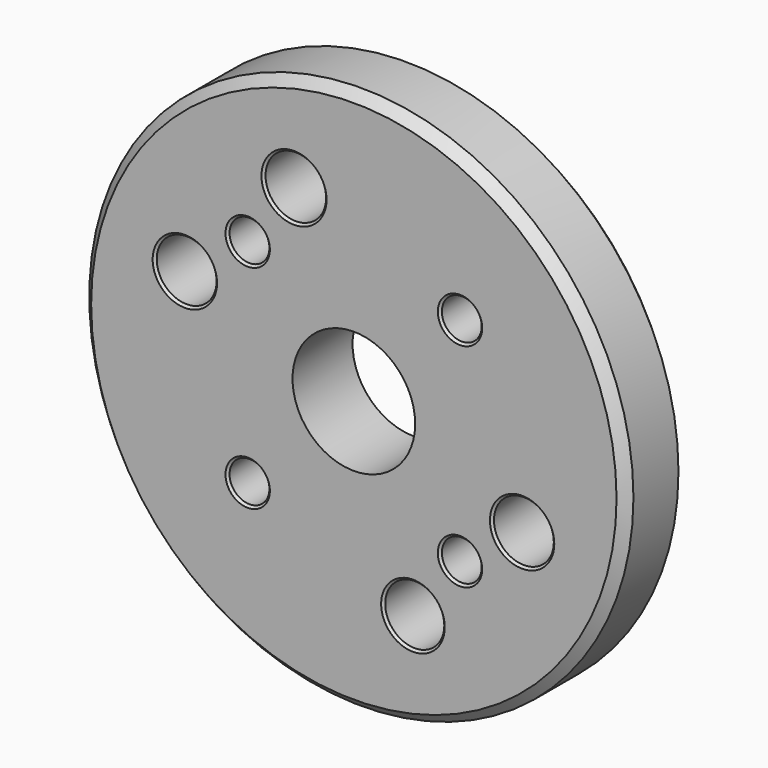
from build123d import *

# Parameters (mm, degrees)
F0_R     = 92.075
F0_R_2   = 20.75
F1_DEPTH = 25.4
F2_R     = 10.125
F2_R_2   = 10.25
F2_R_3   = 10
F3_DEPTH = 25.4
F5_D     = 13.49248
F6_SIZE  = 3.175
F7_SIZE  = 0.762


with BuildPart() as f1:
    # F0 (on Front) → F1 (new body)
    with BuildSketch(Plane.XZ):
        Circle(F0_R)
        Circle(F0_R_2, mode=Mode.SUBTRACT)
    extrude(amount=-F1_DEPTH)

    # F2 (on face) → F3 (cut)
    with BuildSketch(Plane.XZ):
        with Locations((-57.1871926221, 20.125)):
            Circle(F2_R)
        with Locations((-20.25, 57.010415715)):
            Circle(F2_R_2)
        with Locations((56.9371926221, -20.4780090433)):
            Circle(F2_R)
        with Locations((20, -57.3634247583)):
            Circle(F2_R_3)
    extrude(amount=-F3_DEPTH, mode=Mode.SUBTRACT)

    # F5 (through all)
    with Locations(Plane.XZ):
        with Locations((-35.9210244843, 35.9210244843), (35.9210244843, 35.9210244843), (35.9210244843, -35.9210244843), (-35.9210244843, -35.9210244843)):
            Hole(F5_D / 2)

    # F6
    f6_edges = [f1.edges().sort_by_distance(p)[0] for p in [
        (92.075, 12.7, 0),
        (-92.075, 0, 0),
        (-92.075, 25.4, 0),
    ]]
    chamfer(f6_edges, length=F6_SIZE)

    # F7
    f7_edges = [f1.edges().sort_by_distance(p)[0] for p in [
        (-47.062193, 12.7, 20.125),
        (-67.312193, 0, 20.125),
        (-67.312193, 25.4, 20.125),
        (-10, 12.7, 57.010416),
        (-30.5, 0, 57.010416),
        (-30.5, 25.4, 57.010416),
        (67.062193, 12.7, -20.478009),
        (46.812193, 0, -20.478009),
        (46.812193, 25.4, -20.478009),
        (30, 12.7, -57.363425),
        (10, 0, -57.363425),
        (10, 25.4, -57.363425),
        (-42.667264, 0, -35.921024),
        (29.174784, 0, -35.921024),
        (-42.667264, 0, 35.921024),
        (29.174784, 0, 35.921024),
        (-42.667264, 25.4, -35.921024),
        (29.174784, 25.4, -35.921024),
        (-42.667264, 25.4, 35.921024),
        (29.174784, 25.4, 35.921024),
    ]]
    chamfer(f7_edges, length=F7_SIZE)


solid = f1.part
